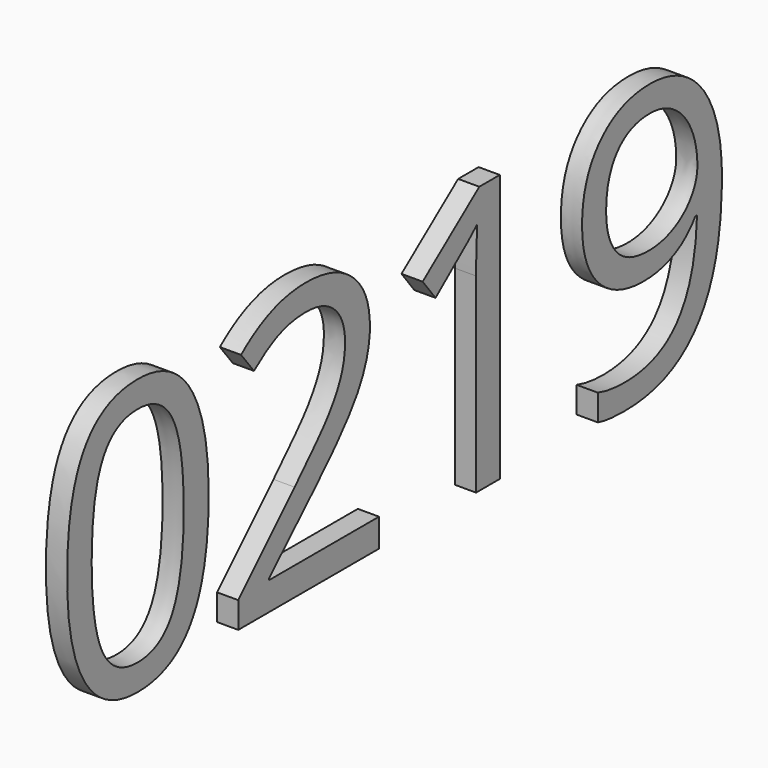
from build123d import *

# Parameters (mm, degrees)
F0_TEXT_SIZE = 10.6264811216
F1_DEPTH     = 0.6


# Not quite as in the source:
# - Text() gives the source's letters only with a copy of the font that has no kerning and outlines rounded to 1/6400 em; it was checked with that copy


with BuildPart() as f1:
    # F0 (on Right) → F1 (new body)
    with BuildSketch(Plane.YZ):
        with Locations((-14.6489944309, 4.5719789341)):
            Text('0219', F0_TEXT_SIZE, font='Open Sans', text_align=(TextAlign.LEFT, TextAlign.BOTTOM))
    extrude(amount=F1_DEPTH)


solid = f1.part
